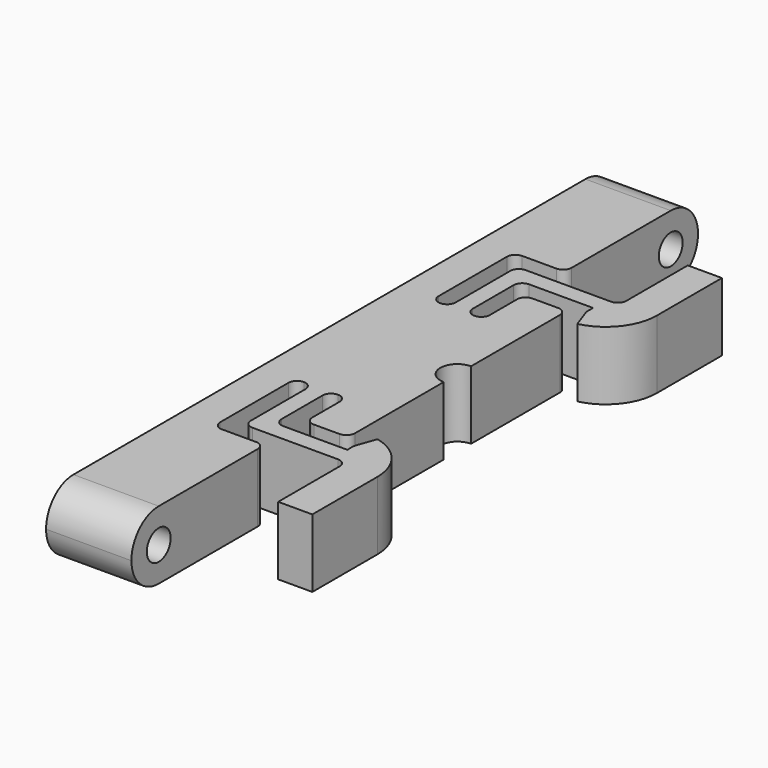
from build123d import *

# Parameters (mm, degrees)
F0_W        = 4
F0_H        = 8
F0_H_2      = 2
F0_W_2      = 5.5
F0_H_3      = 3.5
F1_DEPTH    = 8
F2_R        = 3.99999
F3_T1_DEPTH = 37.8956518578
F4_T1_DEPTH = 21.1532650868
F5_T1_DEPTH = 21.1532650868
F7_DEPTH    = 8
F8_R        = 0.99999
F9_R        = 1.75
F10_DEPTH   = 10


# Not quite as in the source:
# - a fillet or chamfer that OpenCascade refuses, or shapes differently, is made with other operations: its cross-section is extruded or revolved along the edge and cut away or added
# - a fillet or chamfer is up to 0.001 mm smaller than in the source, because OpenCascade refuses the exact size


with BuildPart() as f1:
    # F0 (on Top) → F1 (new body)
    with BuildSketch(Plane.XY):
        Polygon((0, 83), (0, 0), (10, 0), (10, 10), (10, 19.5), (8, 19.5), (4, 19.5), (4, 31.5), (6, 31.5), (8, 31.5), (10, 31.5), (10, 25.5), (15, 25.5), (15, 57.5), (10, 57.5), (10, 51.5), (8, 51.5), (6, 51.5), (4, 51.5), (4, 63.5), (8, 63.5), (10, 63.5), (10, 73), (10, 83), align=None)
        with Locations((20, 67.5)):
            Rectangle(F0_W, F0_H)
        with Locations((20, 62.5)):
            Rectangle(F0_W, F0_H_2)
        with Locations((19.25, 57.75)):
            Rectangle(F0_W_2, F0_H_3)
        with Locations((19.25, 25.25)):
            Rectangle(F0_W_2, F0_H_3)
        with Locations((20, 20.5)):
            Rectangle(F0_W, F0_H_2)
        with Locations((20, 15.5)):
            Rectangle(F0_W, F0_H)
        Polygon((8, 23.5), (8, 21.5), (18, 21.5), (22, 21.5), (22, 23.5), (16.5, 23.5), (15, 23.5), align=None)
        Polygon((6, 21.5), (8, 21.5), (8, 23.5), (8, 25.5), (8, 31.5), (6, 31.5), align=None)
        Polygon((8, 59.5), (8, 61.5), (6, 61.5), (6, 51.5), (8, 51.5), (8, 57.5), align=None)
        Polygon((18, 61.5), (8, 61.5), (8, 59.5), (15, 59.5), (16.5, 59.5), (22, 59.5), (22, 61.5), align=None)
    extrude(amount=F1_DEPTH)

    # F2 (radius 4 in the source; OpenCascade refuses exactly that, so slightly less here)
    f2_edges = [f1.edges().sort_by_distance(p)[0] for p in [
        (5, 83, 8),
        (5, 0, 8),
        (5, 0, 0),
        (5, 83, 0),
    ]]
    fillet(f2_edges, radius=F2_R)

    # F3: fillet of radius 6 on 2 edges, made by hand

    # F3_s2 → F3_t1 (cut)
    with BuildSketch(Plane.XY.offset(-14.9478259289)):
        with BuildLine():
            ThreePointArc((22, 61.9791303716), (20.4158804332, 57.9171111692), (16.5, 56))
            Line((16.5, 56), (22, 56))
            Line((22, 56), (22, 61.9791303716))
        make_face()
        with BuildLine():
            ThreePointArc((22, 21.0208696284), (20.4158804332, 25.0828888308), (16.5, 27))
            Line((16.5, 27), (22, 27))
            Line((22, 27), (22, 21.0208696284))
        make_face()
    extrude(amount=F3_T1_DEPTH, mode=Mode.SUBTRACT)

    # F4: chamfer of 0.5 x 2.5 on 1 edges, made by hand

    # F4_s2 → F4_t1 (cut)
    with BuildSketch(Plane.XY.offset(-6.5766325434)):
        with BuildLine():
            Line((17.379363756, 56.0377654524), (16.466798813, 58.6304434947))
            Line((16.466798813, 58.6304434947), (16.416798813, 58.6304434947))
            ThreePointArc((16.416798813, 58.6304434947), (16.45, 57.3152217474), (16.45, 56))
            Line((16.45, 56), (16.5041666667, 55.9501739136))
            ThreePointArc((16.5041666667, 55.9501739136), (16.9421943049, 56.0029468158), (17.3905817774, 55.9890401407))
            Line((17.3905817774, 55.9890401407), (17.379363756, 56.0377654524))
        make_face()
    extrude(amount=F4_T1_DEPTH, mode=Mode.SUBTRACT)

    # F5: chamfer of 0.5 x 2.5 on 1 edges, made by hand

    # F5_s2 → F5_t1 (cut)
    with BuildSketch(Plane.XY.offset(-6.5766325434)):
        with BuildLine():
            Line((16.466798813, 24.3695565053), (17.379363756, 26.9622345476))
            Line((17.379363756, 26.9622345476), (17.3905817774, 27.0109598593))
            ThreePointArc((17.3905817774, 27.0109598593), (16.9421943049, 26.9970531842), (16.5041666667, 27.0498260864))
            Line((16.5041666667, 27.0498260864), (16.45, 27))
            ThreePointArc((16.45, 27), (16.45, 25.6847782526), (16.416798813, 24.3695565053))
            Line((16.416798813, 24.3695565053), (16.466798813, 24.3695565053))
        make_face()
    extrude(amount=F5_T1_DEPTH, mode=Mode.SUBTRACT)

    # F6 (on face) → F7 (cut)
    with BuildSketch(Plane(origin=(0, 0, 0), x_dir=(1, 0, 0), z_dir=(0, 0, -1))):
        with BuildLine():
            Line((15, -43.5), (15, -39.5))
            ThreePointArc((15, -39.5), (13, -41.5), (15, -43.5))
        make_face()
    extrude(amount=-F7_DEPTH, mode=Mode.SUBTRACT)

    # F8 (radius 1 in the source; OpenCascade refuses exactly that, so slightly less here)
    f8_edges = [f1.edges().sort_by_distance(p)[0] for p in [
        (18, 21.5, 4),
        (6, 21.5, 4),
        (4, 19.5, 4),
        (10, 19.5, 4),
        (8, 23.5, 4),
        (15, 25.5, 4),
        (10, 25.5, 4),
        (8, 31.5, 4),
        (10, 31.5, 4),
        (6, 31.5, 4),
        (4, 31.5, 4),
        (6, 51.5, 4),
        (10, 51.5, 4),
        (18, 61.5, 4),
        (6, 61.5, 4),
        (10, 57.5, 4),
        (15, 57.5, 4),
        (8, 59.5, 4),
        (4, 51.5, 4),
        (8, 51.5, 4),
        (4, 63.5, 4),
        (10, 63.5, 4),
    ]]
    fillet(f8_edges, radius=F8_R)

    # F9 (on face) → F10 (cut)
    with BuildSketch(Plane(origin=(0, 0, 0), x_dir=(0, -1, 0), z_dir=(-1, 0, 0))):
        with Locations((-79, 4)):
            Circle(F9_R)
        with Locations((-4, 4)):
            Circle(F9_R)
    extrude(amount=-F10_DEPTH, mode=Mode.SUBTRACT)


solid = f1.part
